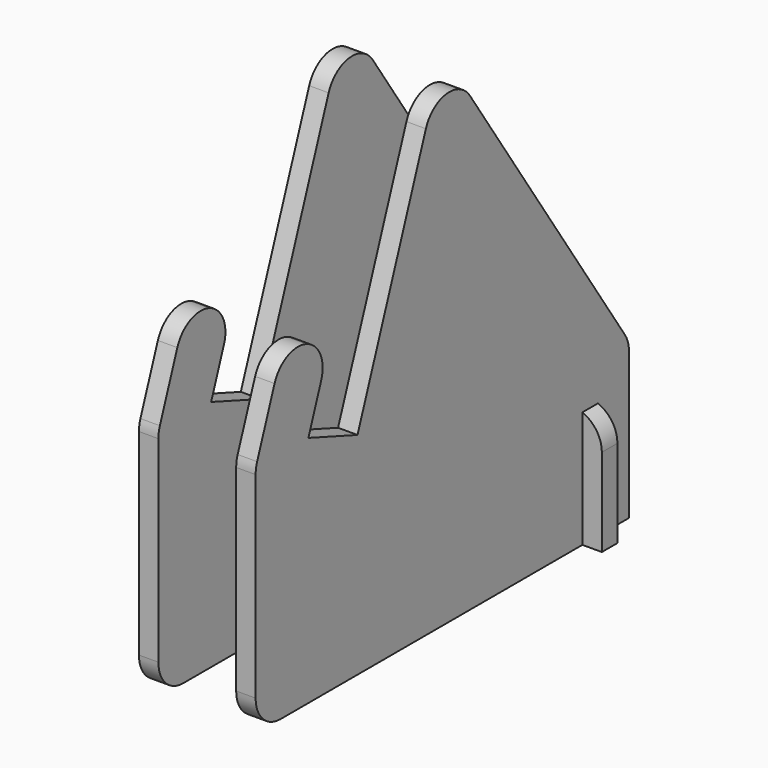
from build123d import *

# Parameters (mm, degrees)
F1_DEPTH      = 3.175
F3_DEPTH      = 3.175
F4_T1_DEPTH   = 7.65370531
F4_T3_DEPTH   = 28.575
F4_T5_DEPTH   = 53.2264881201
F4_T7_DEPTH   = 10.8953858615
F4_2_T1_DEPTH = 26.7214301965
F4_2_T3_DEPTH = 28.575
F6_DEPTH      = 3.175


# Not quite as in the source:
# - a fillet or chamfer that OpenCascade refuses, or shapes differently, is made with other operations: its cross-section is extruded or revolved along the edge and cut away or added


with BuildPart() as f1:
    # F0 (on Right) → F1 (new body)
    with BuildSketch(Plane.YZ):
        Polygon((-6.35, 0), (0, 0), (0, 25.4), (-38.0354831527, 82.1877142469), (-55.4101064336, 34.451329111), (-65.4347473122, 38.1), (-61.0910914919, 50.034096284), (-70.597048836, 53.4939818054), (-76.2, 38.1), (-76.2, 0), (-9.525, 0), (-9.525, 12.7), (-6.35, 12.7), align=None)
    extrude(amount=F1_DEPTH)

    # F4: fillet of radius 5.08 on 6 edges, made by hand

    # F4_s2 → F4_t1 (cut)
    with BuildSketch(Plane.YZ.offset(-2.239352655)):
        with BuildLine():
            ThreePointArc((-75.8936385136, 38.9417212661), (-76.1228233853, 38.0863916805), (-76.2, 37.204258938))
            Line((-76.2, 37.204258938), (-76.2, 38.1))
            Line((-76.2, 38.1), (-75.8936385136, 38.9417212661))
        make_face()
    extrude(amount=F4_T1_DEPTH, mode=Mode.SUBTRACT)

    # F4_s4 → F4_t3 (cut)
    with BuildSketch(Plane.YZ.offset(-12.7)):
        with BuildLine():
            ThreePointArc((-65.8234103224, 51.7565194773), (-69.7077734201, 51.5869245219), (-72.3345111641, 48.7203432918))
            Line((-72.3345111641, 48.7203432918), (-70.597048836, 53.4939818054))
            Line((-70.597048836, 53.4939818054), (-65.8234103224, 51.7565194773))
        make_face()
        with BuildLine():
            ThreePointArc((-62.82855382, 45.2604577704), (-62.9981487755, 49.1448208681), (-65.8647300055, 51.7715586121))
            Line((-65.8647300055, 51.7715586121), (-61.0910914919, 50.034096284))
            Line((-61.0910914919, 50.034096284), (-62.82855382, 45.2604577704))
        make_face()
        with BuildLine():
            ThreePointArc((-76.2, 5.08), (-74.7121024484, 1.4878975516), (-71.12, 0))
            Line((-71.12, 0), (-76.2, 0))
            Line((-76.2, 0), (-76.2, 5.08))
        make_face()
    extrude(amount=F4_T3_DEPTH, mode=Mode.SUBTRACT)

    # F4_s6 → F4_t5 (cut)
    with BuildSketch(Plane.YZ.offset(-25.0257440601)):
        with BuildLine():
            ThreePointArc((-32.4648343865, 73.8706275668), (-37.2964586363, 76.0867843163), (-41.4592065808, 72.7811114378))
            Line((-41.4592065808, 72.7811114378), (-38.0354831527, 82.1877142469))
            Line((-38.0354831527, 82.1877142469), (-32.4648343865, 73.8706275668))
        make_face()
    extrude(amount=F4_T5_DEPTH, mode=Mode.SUBTRACT)

    # F4_s8 → F4_t7 (cut)
    with BuildSketch(Plane.YZ.offset(-3.8601929308)):
        with BuildLine():
            ThreePointArc((0, 23.8559228277), (-0.2195613831, 25.3332638347), (-0.8592663193, 26.6829012848))
            Line((-0.8592663193, 26.6829012848), (0, 25.4))
            Line((0, 25.4), (0, 23.8559228277))
        make_face()
    extrude(amount=F4_T7_DEPTH, mode=Mode.SUBTRACT)


with BuildPart() as f3:
    # F2 (on face) → F3 (new body)
    with BuildSketch(Plane.XZ.offset(6.35)):
        Polygon((3.175, 19.05), (3.175, 12.7), (0, 12.7), (0, 19.05), (-12.7, 19.05), (-12.7, 12.7), (-15.875, 12.7), (-15.875, 19.05), (-19.05, 19.05), (-19.05, 0), (6.35, 0), (6.35, 19.05), align=None)
    extrude(amount=F3_DEPTH)

    # F4#2: fillet of radius 5.08 on 3 edges, made by hand

    # F4_2_s2 → F4_2_t1 (cut)
    with BuildSketch(Plane.XZ.offset(-5.4232150983)):
        with BuildLine():
            ThreePointArc((6.35, 14.3407139607), (5.4821134838, 17.1805202921), (3.175, 19.05))
            Line((3.175, 19.05), (6.35, 19.05))
            Line((6.35, 19.05), (6.35, 14.3407139607))
        make_face()
        with BuildLine():
            ThreePointArc((-15.875, 19.05), (-18.1821134838, 17.1805202921), (-19.05, 14.3407139607))
            Line((-19.05, 14.3407139607), (-19.05, 19.05))
            Line((-19.05, 19.05), (-15.875, 19.05))
        make_face()
    extrude(amount=F4_2_T1_DEPTH, mode=Mode.SUBTRACT)

    # F4_2_s4 → F4_2_t3 (cut)
    with BuildSketch(Plane.XZ.offset(-6.35)):
        with BuildLine():
            ThreePointArc((-13.97, 0), (-17.5621024484, 1.4878975516), (-19.05, 5.08))
            Line((-19.05, 5.08), (-19.05, 0))
            Line((-19.05, 0), (-13.97, 0))
        make_face()
    extrude(amount=F4_2_T3_DEPTH, mode=Mode.SUBTRACT)


with BuildPart() as f6:
    # F5 (on face) → F6 (new body)
    with BuildSketch(Plane(origin=(-12.7, 0, 0), x_dir=(0, -1, 0), z_dir=(-1, 0, 0))):
        with BuildLine():
            Line((75.8936385136, 38.9417212661), (72.3345111641, 48.7203432918))
            ThreePointArc((72.3345111641, 48.7203432918), (69.7177313424, 51.5822679428), (65.844086436, 51.7639943376))
            ThreePointArc((65.844086436, 51.7639943376), (62.9935137558, 49.1348528926), (62.82855382, 45.2604577704))
            Line((62.82855382, 45.2604577704), (65.4347473122, 38.1))
            Line((65.4347473122, 38.1), (55.4101064336, 34.451329111))
            Line((55.4101064336, 34.451329111), (41.4592065808, 72.7811114378))
            ThreePointArc((41.4592065808, 72.7811114378), (37.2964586363, 76.0867843163), (32.4648343865, 73.8706275668))
            Line((32.4648343865, 73.8706275668), (0.8592663193, 26.6829012848))
            ThreePointArc((0.8592663193, 26.6829012848), (0.2195613831, 25.3332638347), (0, 23.8559228277))
            Line((0, 23.8559228277), (0, 0))
            Line((0, 0), (6.35, 0))
            Line((6.35, 0), (6.35, 12.7))
            Line((6.35, 12.7), (6.35, 19.05))
            Line((6.35, 19.05), (9.525, 19.05))
            Line((9.525, 19.05), (9.525, 12.7))
            Line((9.525, 12.7), (9.525, 0))
            Line((9.525, 0), (71.12, 0))
            ThreePointArc((71.12, 0), (74.7121024484, 1.4878975516), (76.2, 5.08))
            Line((76.2, 5.08), (76.2, 37.204258938))
            ThreePointArc((76.2, 37.204258938), (76.1228233853, 38.0863916805), (75.8936385136, 38.9417212661))
        make_face()
    extrude(amount=F6_DEPTH)


solid = Compound([f1.part, f3.part, f6.part])
